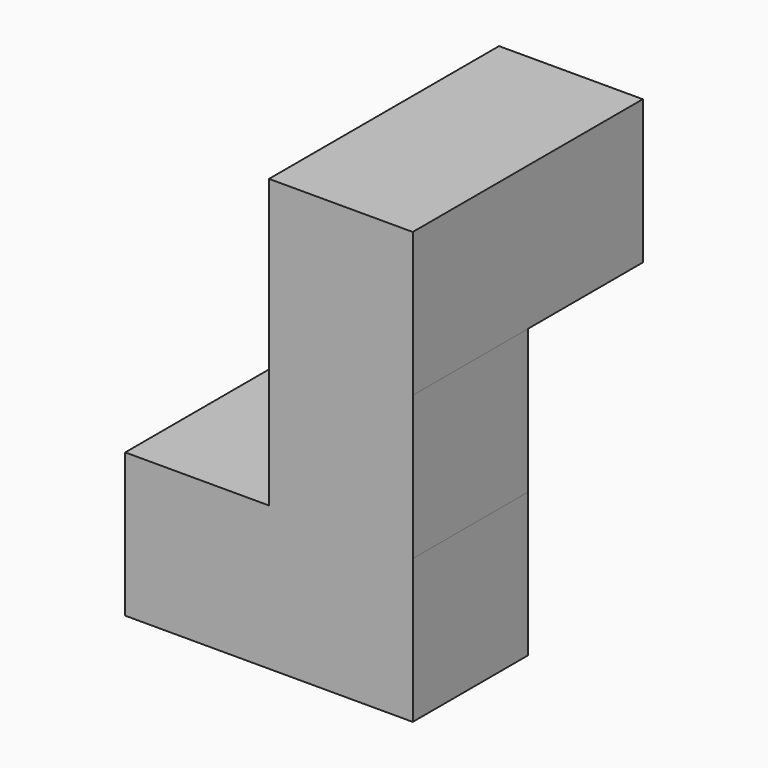
from build123d import *

# Parameters (mm, degrees)
F1_DEPTH = 12.7
F0_W     = 12.7
F0_H     = 12.7
F2_DEPTH = 12.7


# Not quite as in the source:
# - ends of sketch curves that miss each other by under 0.0002 mm in the source are joined


with BuildPart() as f1:
    # F0 (on Front) → F1 (new body)
    with BuildSketch(Plane.XZ):
        Polygon((-28.6124870216, 26.0709726285), (-41.3124847398, 26.0709726285), (-41.3124847398, 13.3709726285), (-28.6124870216, 13.3709749104), align=None)
        Polygon((-41.3124847398, 38.7709726285), (-41.3124847398, 26.0709726285), (-28.6124870216, 26.0709726285), (-28.6124847398, 38.7709726285), align=None)
    extrude(amount=F1_DEPTH)

    # F0 (on Front) → F2 (join, symmetric)
    with BuildSketch(Plane.XZ):
        with Locations((-47.6624847398, 19.7209726285)):
            Rectangle(F0_W, F0_H)
        with Locations((-34.9624847398, 45.1209726285)):
            Rectangle(F0_W, F0_H)
    extrude(amount=F2_DEPTH, both=True)


solid = f1.part
